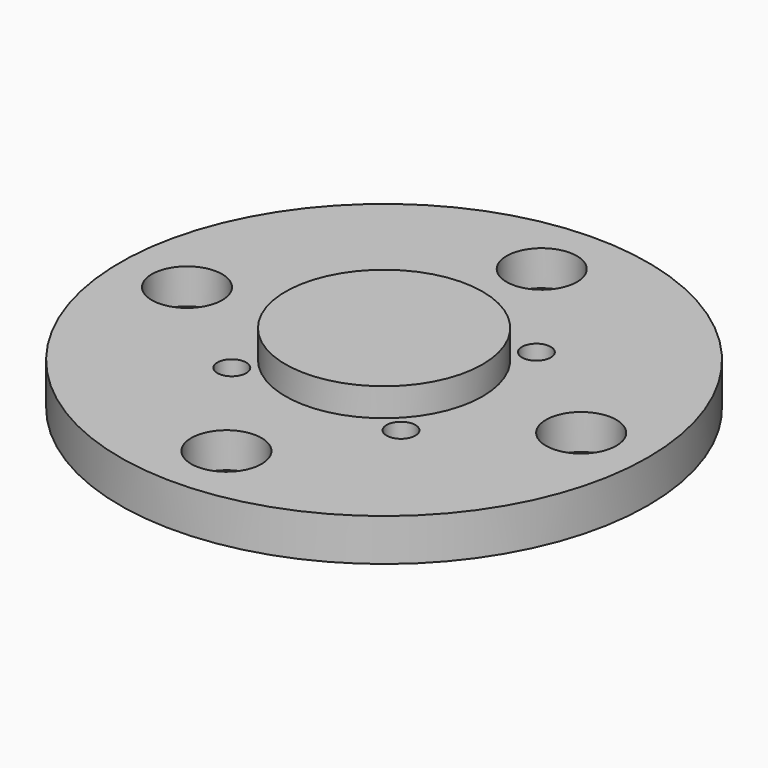
from build123d import *

# Parameters (mm, degrees)
F0_R            = 37.5
F1_DEPTH        = 10
F2_R            = 37.5
F2_R_2          = 14
F3_DEPTH        = 4
F5_D            = 5
F5_CBORE_D      = 10
F5_CBORE_DEPTH  = 5
F5_COPIES_COUNT = 4
F7_D            = 4.1
F7_COPIES_COUNT = 4


# Not quite as in the source:
# - a pattern or mirror of a feature is missing from the dataset's text; its kind, count and spacing are read off the source's solid
# - a feature names something its author has since deleted; it is built from what else it names


with BuildPart() as f1:
    # F0 (on Top) → F1 (new body)
    with BuildSketch(Plane.XY):
        Circle(F0_R)
    extrude(amount=F1_DEPTH)

    # F2 (on face) → F3 (cut)
    with BuildSketch(Plane.XY.offset(10)):
        Circle(F2_R)
        Circle(F2_R_2, mode=Mode.SUBTRACT)
    extrude(amount=-F3_DEPTH, mode=Mode.SUBTRACT)

    # F5 (through all)
    with Locations(Plane.XY.offset(6)):
        with Locations((0, 28)):
            f5 = CounterBoreHole(F5_D / 2, F5_CBORE_D / 2, F5_CBORE_DEPTH)

    # F5_copies: F5 ×4 about axis
    f5_copies_axis = Axis((0, 0, 0), (0, 0, 1))
    for i in range(1, F5_COPIES_COUNT):
        add(f5.rotate(f5_copies_axis, i * 360 / F5_COPIES_COUNT), mode=Mode.SUBTRACT)

    # F7 (through all)
    with Locations(Plane(origin=(0, 0, 0), x_dir=(1, 0, 0), z_dir=(0, 0, -1))):
        with Locations((-12.0208152802, 12.0208152802)):
            f7 = Hole(F7_D / 2)

    # F7_copies: F7 ×4 about axis
    f7_copies_axis = Axis((0, 0, 0), (0, 0, 1))
    for i in range(1, F7_COPIES_COUNT):
        add(f7.rotate(f7_copies_axis, i * 360 / F7_COPIES_COUNT), mode=Mode.SUBTRACT)


solid = f1.part
